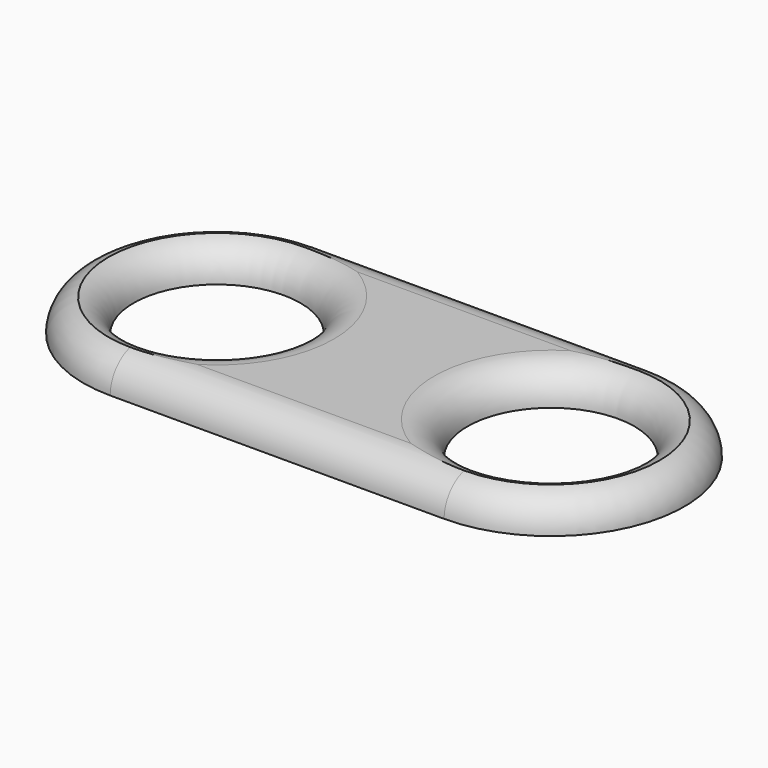
from build123d import *

# Parameters (mm, degrees)
F0_R         = 2.5
F1_DEPTH     = 1
F2_T1_DEPTH  = 10
F2_T4_ANGLE  = 180
F2_T10_ANGLE = 180


# Not quite as in the source:
# - a fillet or chamfer that OpenCascade refuses, or shapes differently, is made with other operations: its cross-section is extruded or revolved along the edge and cut away or added


with BuildPart() as f1:
    # F0 (on Top) → F1 (new body)
    with BuildSketch(Plane.XY):
        with BuildLine():
            Line((5, 4), (-5, 4))
            ThreePointArc((-5, 4), (-9, 0), (-5, -4))
            Line((-5, -4), (5, -4))
            ThreePointArc((5, -4), (9, 0), (5, 4))
        make_face()
        with Locations((-5, 0)):
            Circle(F0_R, mode=Mode.SUBTRACT)
        with Locations((5, 0)):
            Circle(F0_R, mode=Mode.SUBTRACT)
    extrude(amount=F1_DEPTH)

    # F2: fillet of radius 1 on 3 edges, made by hand

    # F2_s2 → F2_t1 (cut)
    with BuildSketch(Plane.YZ.offset(-5)):
        with BuildLine():
            ThreePointArc((4, 0), (3.7071067812, 0.7071067812), (3, 1))
            Line((3, 1), (4, 1))
            Line((4, 1), (4, 0))
        make_face()
        with BuildLine():
            ThreePointArc((-4, 0), (-3.7071067812, 0.7071067812), (-3, 1))
            Line((-3, 1), (-4, 1))
            Line((-4, 1), (-4, 0))
        make_face()
    extrude(amount=F2_T1_DEPTH, mode=Mode.SUBTRACT)

    # F2_s3 → F2_t4 (revolve, cut)
    with BuildSketch(Plane.YZ.offset(-5)):
        with BuildLine():
            ThreePointArc((4, 0), (3.7071067812, 0.7071067812), (3, 1))
            Line((3, 1), (4, 1))
            Line((4, 1), (4, 0))
        make_face()
    revolve(axis=Axis((-5, 0, 1), (0, 0, 1)), revolution_arc=F2_T4_ANGLE, mode=Mode.SUBTRACT)

    # F2_s5 → F2_t6 (revolve, cut)
    with BuildSketch(Plane.XZ):
        with BuildLine():
            ThreePointArc((-2.5, 0), (-2.2071067812, 0.7071067812), (-1.5, 1))
            Line((-1.5, 1), (-2.5, 1))
            Line((-2.5, 1), (-2.5, 0))
        make_face()
    revolve(axis=Axis((-5, 0, 1), (0, 0, 1)), mode=Mode.SUBTRACT)

    # F2_s7 → F2_t8 (revolve, cut)
    with BuildSketch(Plane.XZ):
        with BuildLine():
            ThreePointArc((7.5, 0), (7.7928932188, 0.7071067812), (8.5, 1))
            Line((8.5, 1), (7.5, 1))
            Line((7.5, 1), (7.5, 0))
        make_face()
    revolve(axis=Axis((5, 0, 1), (0, 0, 1)), mode=Mode.SUBTRACT)

    # F2_s9 → F2_t10 (revolve, cut)
    with BuildSketch(Plane.YZ.offset(5)):
        with BuildLine():
            ThreePointArc((-4, 0), (-3.7071067812, 0.7071067812), (-3, 1))
            Line((-3, 1), (-4, 1))
            Line((-4, 1), (-4, 0))
        make_face()
    revolve(axis=Axis((5, 0, 1), (0, 0, 1)), revolution_arc=F2_T10_ANGLE, mode=Mode.SUBTRACT)


solid = f1.part
